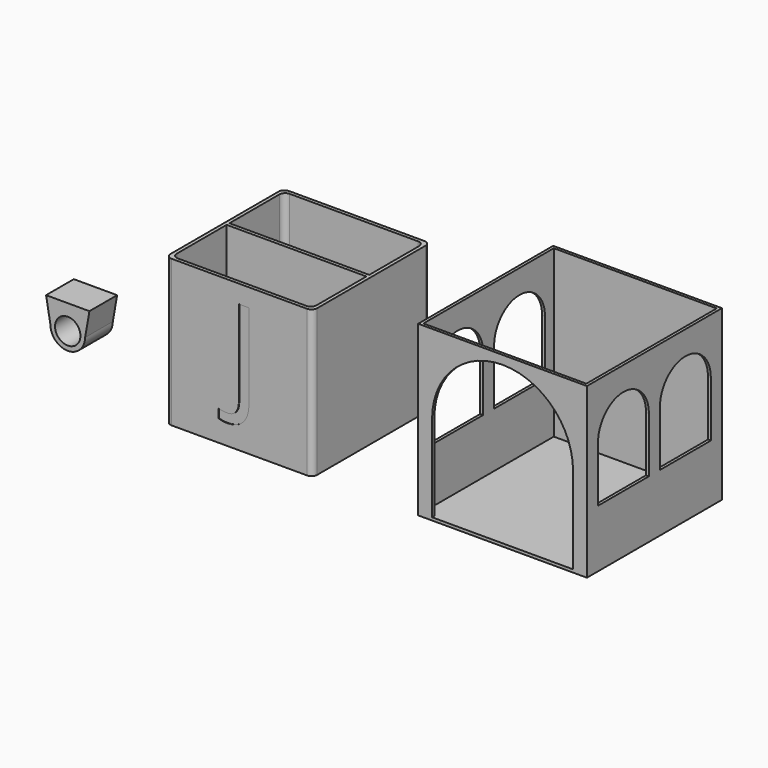
from build123d import *

# Parameters (mm, degrees)
F2_R          = 2.5
F4_W          = 127
F4_H          = 127
F5_DEPTH      = 127
F6_T          = -3
F7_R          = 5
F8_R          = 5
F9_W          = 121
F9_H          = 3
F10_DEPTH     = 124
F11_TEXT_SIZE = 104.1666666667
F12_DEPTH     = 0.5
F13_W         = 146.05
F13_H         = 146.05
F14_DEPTH     = 146.05
F15_T         = -2.5
F17_DEPTH     = 25
F19_DEPTH     = 168
F20_R         = 11
F21_DEPTH     = 30


# Not quite as in the source:
# - Text() gives the source's letters only with a copy of the font that has no kerning and outlines rounded to 1/6400 em; it was checked with that copy


with BuildPart() as f1:
    # F0 (on Front) → F1 (revolve)
    with BuildSketch(Plane.XZ):
        Polygon((-133.35, 228.6), (-93.04165221, 0), (0, 0), (0, 10), (-84.8049220171, 10), (-123.35, 228.6), align=None)
    revolve(axis=Axis((0, 0, 5), (0, 0, -1)))

    # F2
    f2_edges = [f1.edges().sort_by_distance(p)[0] for p in [
        (93.041652, 0, 0),
        (133.35, 0, 228.6),
        (123.35, 0, 228.6),
    ]]
    fillet(f2_edges, radius=F2_R)


with BuildPart() as f5:
    # F4 (on Top) → F5 (new body)
    with BuildSketch(Plane.XY):
        with Locations((-47.6122590086, 0.4123076797)):
            Rectangle(F4_W, F4_H)
    extrude(amount=F5_DEPTH)

    # F6
    f6_openings = [f5.faces().sort_by_distance(p)[0] for p in [
        (-47.612259, 0.412308, 127),
    ]]
    offset(amount=F6_T, openings=f6_openings)

    # F7
    f7_edges = [f5.edges().sort_by_distance(p)[0] for p in [
        (12.887741, 60.912308, 65),
        (-108.112259, 60.912308, 65),
        (12.887741, -60.087692, 65),
        (-108.112259, -60.087692, 65),
    ]]
    fillet(f7_edges, radius=F7_R)

    # F8
    f8_edges = [f5.edges().sort_by_distance(p)[0] for p in [
        (-111.112259, -63.087692, 63.5),
        (15.887741, -63.087692, 63.5),
        (-111.112259, 63.912308, 63.5),
        (15.887741, 63.912308, 63.5),
    ]]
    fillet(f8_edges, radius=F8_R)

    # F9 (on face) → F10 (join)
    with BuildSketch(Plane.XY.offset(3)):
        with Locations((-47.6122590086, 0.4123076797)):
            Rectangle(F9_W, F9_H)
    extrude(amount=F10_DEPTH)

    # F11 (on face) → F12 (cut)
    with BuildSketch(Plane.XZ.offset(63.0876923203)):
        with Locations((-57.6122590086, 37)):
            Text('J', F11_TEXT_SIZE, font='Open Sans', text_align=(TextAlign.LEFT, TextAlign.BOTTOM))
    extrude(amount=-F12_DEPTH, mode=Mode.SUBTRACT)


with BuildPart() as f14:
    # F13 (on Top) → F14 (new body)
    with BuildSketch(Plane.XY):
        with Locations((179.286496985, 11.1893585762)):
            Rectangle(F13_W, F13_H)
    extrude(amount=F14_DEPTH)

    # F15
    f15_openings = [f14.faces().sort_by_distance(p)[0] for p in [
        (179.286497, 11.189359, 146.05),
    ]]
    offset(amount=F15_T, openings=f15_openings)

    # F16 (on face) → F17 (cut)
    with BuildSketch(Plane.XZ.offset(61.8356414238)):
        with BuildLine():
            Line((118.261496985, 77.5), (118.261496985, 2.5))
            Line((118.261496985, 2.5), (240.311496985, 2.5))
            Line((240.311496985, 2.5), (240.311496985, 77.5))
            ThreePointArc((240.311496985, 77.5), (179.286496985, 138.525), (118.261496985, 77.5))
        make_face()
    extrude(amount=-F17_DEPTH, mode=Mode.SUBTRACT)

    # F18 (on face) → F19 (cut)
    with BuildSketch(Plane.YZ.offset(252.311496985)):
        with BuildLine():
            Line((-49.8356414238, 98), (-49.8356414238, 50))
            Line((-49.8356414238, 50), (5.1893585762, 50))
            Line((5.1893585762, 50), (5.1893585762, 98))
            ThreePointArc((5.1893585762, 98), (-22.3231414238, 125.5125), (-49.8356414238, 98))
        make_face()
        with BuildLine():
            ThreePointArc((72.2143585762, 98), (44.7018585762, 125.5125), (17.1893585762, 98))
            Line((17.1893585762, 98), (17.1893585762, 50))
            Line((17.1893585762, 50), (72.2143585762, 50))
            Line((72.2143585762, 50), (72.2143585762, 98))
        make_face()
    extrude(amount=-F19_DEPTH, mode=Mode.SUBTRACT)


with BuildPart() as f21:
    # F20 (on Front) → F21 (new body)
    with BuildSketch(Plane.XZ):
        with BuildLine():
            Line((-241.2888536627, 41.8613124568), (-237.5295627044, 20.5413139904))
            ThreePointArc((-237.5295627044, 20.5413139904), (-222.5295627044, 5.5413139904), (-207.5295627044, 20.5413139904))
            Line((-207.5295627044, 20.5413139904), (-203.7702717461, 41.8613124568))
            Line((-203.7702717461, 41.8613124568), (-241.2888536627, 41.8613124568))
        make_face()
        with Locations((-222.5295627044, 20.5413139904)):
            Circle(F20_R, mode=Mode.SUBTRACT)
    extrude(amount=F21_DEPTH)


solid = Compound([f5.part, f14.part, f21.part])
